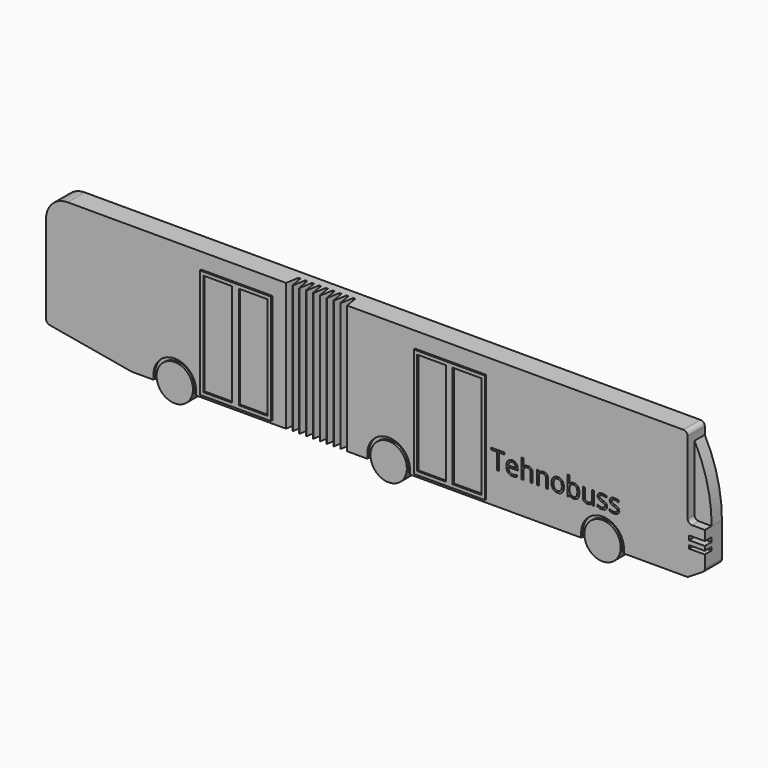
from build123d import *

# Parameters (mm, degrees)
F1_DEPTH      = 5
F4_DEPTH      = 0.5
F5_DEPTH      = 5
F6_W          = 0.5
F6_H          = 30
F7_DEPTH      = 3
F8_SIZE2      = 2.99999
F8_SIZE       = 0.49999
F8_2_SIZE2    = 2.99999
F8_2_SIZE     = 0.49999
F8_3_SIZE2    = 2.99999
F8_3_SIZE     = 0.49999
F8_4_SIZE2    = 2.99999
F8_4_SIZE     = 0.49999
F8_5_SIZE2    = 2.99999
F8_5_SIZE     = 0.49999
F8_6_SIZE2    = 2.99999
F8_6_SIZE     = 0.49999
F8_7_SIZE2    = 2.99999
F8_7_SIZE     = 0.49999
F8_8_SIZE2    = 2.99999
F8_8_SIZE     = 0.49999
F8_9_SIZE2    = 2.99999
F8_9_SIZE     = 0.49999
F8_10_SIZE2   = 2.99999
F8_10_SIZE    = 0.49999
F10_W         = 16.6
F10_H         = 25.6
F10_W_2       = 1.6
F10_H_2       = 24
F11_DEPTH     = 0.4
F12_TEXT_SIZE = 5.9047853364
F13_DEPTH     = 2
F14_W         = 3.7
F14_H         = 1
F14_H_2       = 0.75
F15_DEPTH     = 2
F16_R         = 1


# Not quite as in the source:
# - two fillets or chamfers of one size are made in one step
# - a fillet or chamfer is up to 0.001 mm smaller than in the source, because OpenCascade refuses the exact size
# - a feature of the source that left no trace in its solid (it failed there, or was rolled back) is left out
# - Text() gives the source's letters only with a copy of the font that has no kerning and outlines rounded to 1/6400 em; it was checked with that copy


with BuildPart() as f1:
    # F0 (on Front) → F1 (new body)
    with BuildSketch(Plane.XZ):
        with BuildLine():
            Line((75, 12.2480768093), (75, 15))
            Line((75, 15), (-70, 15))
            ThreePointArc((-70, 15), (-73.5355339059, 13.5355339059), (-75, 10))
            Line((-75, 10), (-75, -11.5))
            Line((-75, -11.5), (-55, -15))
            Line((-55, -15), (75, -15))
            Line((75, -15), (75, 12.2480768093))
        make_face()
        with BuildLine():
            ThreePointArc((79, -4), (77.9852909359, 4.3666002653), (75, 12.2480768093))
            Line((75, 12.2480768093), (75, -15))
            Line((75, -15), (79, -12.5))
            Line((79, -12.5), (79, -4))
        make_face()
    extrude(amount=F1_DEPTH)

    # F3 (on face) → F4 (cut)
    with BuildSketch(Plane.XZ.offset(5)):
        with BuildLine():
            ThreePointArc((-49.0438377664, -15), (-45.416706716, -9.7799359531), (-40.6631598559, -14))
            ThreePointArc((-40.6631598559, -14), (-40.6930958091, -14.50354686), (-40.7824819455, -15))
            Line((-40.7824819455, -15), (-39.9131598559, -15))
            Line((-39.9131598559, -15), (-39.9131598559, -14))
            ThreePointArc((-39.9131598559, -14), (-44.9131598559, -9), (-49.9131598559, -14))
            Line((-49.9131598559, -14), (-49.9131598559, -15))
            Line((-49.9131598559, -15), (-49.0438377664, -15))
        make_face()
        with BuildLine():
            ThreePointArc((-40.7824819455, -15), (-40.6930958091, -14.50354686), (-40.6631598559, -14))
            ThreePointArc((-40.6631598559, -14), (-45.416706716, -9.7799359531), (-49.0438377664, -15))
            Line((-49.0438377664, -15), (-40.7824819455, -15))
        make_face()
        with BuildLine():
            Line((50.0868401441, -14), (50.0868401441, -15))
            Line((50.0868401441, -15), (50.9561622336, -15))
            ThreePointArc((50.9561622336, -15), (54.583293284, -9.7799359531), (59.3368401441, -14))
            ThreePointArc((59.3368401441, -14), (59.3069041909, -14.50354686), (59.2175180545, -15))
            Line((59.2175180545, -15), (60.0868401441, -15))
            Line((60.0868401441, -15), (60.0868401441, -14))
            ThreePointArc((60.0868401441, -14), (55.0868401441, -9), (50.0868401441, -14))
        make_face()
        with BuildLine():
            ThreePointArc((59.3368401441, -14), (54.583293284, -9.7799359531), (50.9561622336, -15))
            Line((50.9561622336, -15), (59.2175180545, -15))
            ThreePointArc((59.2175180545, -15), (59.3069041909, -14.50354686), (59.3368401441, -14))
        make_face()
        with BuildLine():
            Line((0.0868401441, -14), (0.0868401441, -15))
            Line((0.0868401441, -15), (0.9561622336, -15))
            ThreePointArc((0.9561622336, -15), (4.583293284, -9.7799359531), (9.3368401441, -14))
            ThreePointArc((9.3368401441, -14), (9.3069041909, -14.50354686), (9.2175180545, -15))
            Line((9.2175180545, -15), (10.0868401441, -15))
            Line((10.0868401441, -15), (10.0868401441, -14))
            ThreePointArc((10.0868401441, -14), (5.0868401441, -9), (0.0868401441, -14))
        make_face()
        with BuildLine():
            ThreePointArc((9.3368401441, -14), (4.583293284, -9.7799359531), (0.9561622336, -15))
            Line((0.9561622336, -15), (9.2175180545, -15))
            ThreePointArc((9.2175180545, -15), (9.3069041909, -14.50354686), (9.3368401441, -14))
        make_face()
    extrude(amount=-F4_DEPTH, mode=Mode.SUBTRACT)

    # F3 (on face) → F5 (join)
    with BuildSketch(Plane.XZ.offset(5)):
        with BuildLine():
            Line((-40.7824819455, -15), (-49.0438377664, -15))
            ThreePointArc((-49.0438377664, -15), (-44.9131598559, -18.25), (-40.7824819455, -15))
        make_face()
        with BuildLine():
            ThreePointArc((-40.7824819455, -15), (-40.6930958091, -14.50354686), (-40.6631598559, -14))
            ThreePointArc((-40.6631598559, -14), (-45.416706716, -9.7799359531), (-49.0438377664, -15))
            Line((-49.0438377664, -15), (-40.7824819455, -15))
        make_face()
        with BuildLine():
            Line((9.2175180545, -15), (0.9561622336, -15))
            ThreePointArc((0.9561622336, -15), (5.0868401441, -18.25), (9.2175180545, -15))
        make_face()
        with BuildLine():
            ThreePointArc((9.3368401441, -14), (4.583293284, -9.7799359531), (0.9561622336, -15))
            Line((0.9561622336, -15), (9.2175180545, -15))
            ThreePointArc((9.2175180545, -15), (9.3069041909, -14.50354686), (9.3368401441, -14))
        make_face()
        with BuildLine():
            Line((59.2175180545, -15), (50.9561622336, -15))
            ThreePointArc((50.9561622336, -15), (55.0868401441, -18.25), (59.2175180545, -15))
        make_face()
        with BuildLine():
            ThreePointArc((59.3368401441, -14), (54.583293284, -9.7799359531), (50.9561622336, -15))
            Line((50.9561622336, -15), (59.2175180545, -15))
            ThreePointArc((59.2175180545, -15), (59.3069041909, -14.50354686), (59.3368401441, -14))
        make_face()
    extrude(amount=-F5_DEPTH)

    # F6 (on face) → F7 (cut)
    with BuildSketch(Plane.XZ.offset(5)):
        with Locations((-18.1631598559, 0)):
            Rectangle(F6_W, F6_H)
        with Locations((-16.5631598559, 0)):
            Rectangle(F6_W, F6_H)
        with Locations((-14.9631598559, 0)):
            Rectangle(F6_W, F6_H)
        with Locations((-13.3631598559, 0)):
            Rectangle(F6_W, F6_H)
        with Locations((-11.7631598559, 0)):
            Rectangle(F6_W, F6_H)
        with Locations((-10.1631598559, 0)):
            Rectangle(F6_W, F6_H)
        with Locations((-8.5631598559, 0)):
            Rectangle(F6_W, F6_H)
        with Locations((-6.9631598559, 0)):
            Rectangle(F6_W, F6_H)
        with Locations((-5.3631598559, 0)):
            Rectangle(F6_W, F6_H)
    extrude(amount=-F7_DEPTH, mode=Mode.SUBTRACT)

    # F8 (size 0.5 and 3 in the source; OpenCascade refuses exactly that, so slightly less here)
    f8_edges = [f1.edges().sort_by_distance(p)[0] for p in [
        (-7.21316, -5, 0),
        (-8.31316, -5, 0),
    ]]
    f8_side = f1.faces().sort_by_distance((-7.76316, -5, 0))[0]
    chamfer(f8_edges, length=F8_SIZE, length2=F8_SIZE2, reference=f8_side)

    # F8#2 (size 0.5 and 3 in the source; OpenCascade refuses exactly that, so slightly less here)
    f8_2_edges = [f1.edges().sort_by_distance(p)[0] for p in [
        (-16.81316, -5, 0),
        (-17.91316, -5, 0),
    ]]
    f8_2_side = f1.faces().sort_by_distance((-17.36316, -5, 0))[0]
    chamfer(f8_2_edges, length=F8_2_SIZE, length2=F8_2_SIZE2, reference=f8_2_side)

    # F8#3 (size 0.5 and 3 in the source; OpenCascade refuses exactly that, so slightly less here)
    f8_3_edges = [f1.edges().sort_by_distance(p)[0] for p in [
        (-10.41316, -5, 0),
        (-11.51316, -5, 0),
    ]]
    f8_3_side = f1.faces().sort_by_distance((-10.96316, -5, 0))[0]
    chamfer(f8_3_edges, length=F8_3_SIZE, length2=F8_3_SIZE2, reference=f8_3_side)

    # F8#4 (size 0.5 and 3 in the source; OpenCascade refuses exactly that, so slightly less here)
    f8_4_edges = [f1.edges().sort_by_distance(p)[0] for p in [
        (-5.61316, -5, 0),
        (-6.71316, -5, 0),
    ]]
    f8_4_side = f1.faces().sort_by_distance((-6.16316, -5, 0))[0]
    chamfer(f8_4_edges, length=F8_4_SIZE, length2=F8_4_SIZE2, reference=f8_4_side)

    # F8#5 (size 0.5 and 3 in the source; OpenCascade refuses exactly that, so slightly less here)
    f8_5_edges = [f1.edges().sort_by_distance(p)[0] for p in [
        (-15.21316, -5, 0),
        (-16.31316, -5, 0),
    ]]
    f8_5_side = f1.faces().sort_by_distance((-15.76316, -5, 0))[0]
    chamfer(f8_5_edges, length=F8_5_SIZE, length2=F8_5_SIZE2, reference=f8_5_side)

    # F8#6 (size 0.5 and 3 in the source; OpenCascade refuses exactly that, so slightly less here)
    f8_6_edges = [f1.edges().sort_by_distance(p)[0] for p in [
        (-13.61316, -5, 0),
        (-14.71316, -5, 0),
    ]]
    f8_6_side = f1.faces().sort_by_distance((-14.16316, -5, 0))[0]
    chamfer(f8_6_edges, length=F8_6_SIZE, length2=F8_6_SIZE2, reference=f8_6_side)

    # F8#7 (size 0.5 and 3 in the source; OpenCascade refuses exactly that, so slightly less here)
    f8_7_edges = [f1.edges().sort_by_distance(p)[0] for p in [
        (-12.01316, -5, 0),
        (-13.11316, -5, 0),
    ]]
    f8_7_side = f1.faces().sort_by_distance((-12.56316, -5, 0))[0]
    chamfer(f8_7_edges, length=F8_7_SIZE, length2=F8_7_SIZE2, reference=f8_7_side)

    # F8#8 (size 0.5 and 3 in the source; OpenCascade refuses exactly that, so slightly less here)
    f8_8_edges = [f1.edges().sort_by_distance(p)[0] for p in [
        (-8.81316, -5, 0),
        (-9.91316, -5, 0),
    ]]
    f8_8_side = f1.faces().sort_by_distance((-9.36316, -5, 0))[0]
    chamfer(f8_8_edges, length=F8_8_SIZE, length2=F8_8_SIZE2, reference=f8_8_side)

    # F8#9 (size 0.5 and 3 in the source; OpenCascade refuses exactly that, so slightly less here)
    f8_9_edges = [f1.edges().sort_by_distance(p)[0] for p in [
        (-5.11316, -5, 0),
    ]]
    f8_9_side = f1.faces().sort_by_distance((36.594543, -5, 0.406106))[0]
    chamfer(f8_9_edges, length=F8_9_SIZE, length2=F8_9_SIZE2, reference=f8_9_side)

    # F8#10 (size 0.5 and 3 in the source; OpenCascade refuses exactly that, so slightly less here)
    f8_10_edges = [f1.edges().sort_by_distance(p)[0] for p in [
        (-18.41316, -5, 0),
    ]]
    f8_10_side = f1.faces().sort_by_distance((-46.200116, -5, 0.635042))[0]
    chamfer(f8_10_edges, length=F8_10_SIZE, length2=F8_10_SIZE2, reference=f8_10_side)

    # F10 (on face) → F11 (join)
    with BuildSketch(Plane.XZ.offset(5)):
        with Locations((-30.4131598559, -1.5)):
            Rectangle(F10_W, F10_H)
        Polygon((-37.9131598559, -13.5), (-37.9131598559, 10.5), (-31.2131598559, 10.5), (-29.6131598559, 10.5), (-22.9131598559, 10.5), (-22.9131598559, -13.5), (-29.6131598559, -13.5), (-31.2131598559, -13.5), align=None, mode=Mode.SUBTRACT)
        with Locations((19.5868401441, -1.5)):
            Rectangle(F10_W, F10_H)
        Polygon((18.7868401441, -13.5), (12.0868401441, -13.5), (12.0868401441, 10.5), (18.7868401441, 10.5), (20.3868401441, 10.5), (27.0868401441, 10.5), (27.0868401441, -13.5), (20.3868401441, -13.5), align=None, mode=Mode.SUBTRACT)
        with Locations((-30.4131598559, -1.5)):
            Rectangle(F10_W_2, F10_H_2)
        with Locations((19.5868401441, -1.5)):
            Rectangle(F10_W_2, F10_H_2)
    extrude(amount=F11_DEPTH)

    # F12 (on face) → F13 (cut)
    with BuildSketch(Plane.XZ.offset(5)):
        with Locations((29, -7.5)):
            Text('Tehnobuss', F12_TEXT_SIZE, font='Open Sans', text_align=(TextAlign.LEFT, TextAlign.BOTTOM))
    extrude(amount=-F13_DEPTH, mode=Mode.SUBTRACT)

    # F14 (on face) → F15 (cut)
    with BuildSketch(Plane.XZ.offset(5)):
        with BuildLine():
            ThreePointArc((79, -4), (78.0624426605, 4.0467384697), (75.3, 11.6623752988))
            Line((75.3, 11.6623752988), (75.3, -4))
            Line((75.3, -4), (79, -4))
        make_face()
        with Locations((77.15, -6.8)):
            Rectangle(F14_W, F14_H)
        with Locations((77.15, -8.675)):
            Rectangle(F14_W, F14_H_2)
        with BuildLine():
            Line((75.3, -4), (75.3, 11.6623752988))
            ThreePointArc((75.3, 11.6623752988), (75.1513765597, 11.9559311366), (75, 12.2480768093))
            Line((75, 12.2480768093), (75, -4))
            Line((75, -4), (75.3, -4))
        make_face()
    extrude(amount=-F15_DEPTH, mode=Mode.SUBTRACT)

    # F16
    f16_edges = [f1.edges().sort_by_distance(p)[0] for p in [
        (75, -4, -4),
        (75, -2.5, 15),
        (75, -2.5, -15),
        (79, -2.5, -12.5),
        (-55, -2.5, -15),
        (-75, -2.5, -11.5),
    ]]
    fillet(f16_edges, radius=F16_R)


solid = f1.part
